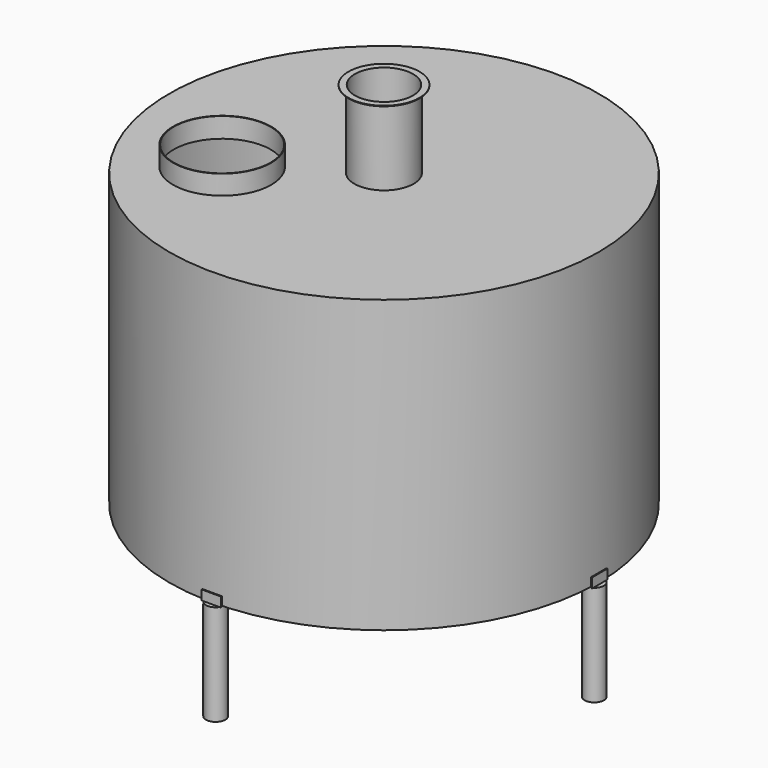
from build123d import *

# Parameters (mm, degrees)
F0_R      = 1106.75
F0_R_2    = 1103.75
F1_DEPTH  = 1500
F2_R      = 1103.75
F3_DEPTH  = 3
F4_R      = 1103.75
F4_R_2    = 250
F4_R_3    = 150
F5_DEPTH  = 3
F6_R      = 253
F6_R_2    = 250
F7_DEPTH  = 100
F8_R      = 153
F8_R_2    = 150
F9_DEPTH  = 400
F10_R     = 183
F10_R_2   = 150
F11_DEPTH = 3
F13_W     = 100
F13_H     = 50
F14_DEPTH = 5
F15_W     = 100
F15_H     = 5
F16_DEPTH = 50
F18_W     = 100
F18_H     = 50
F19_DEPTH = 5
F20_W     = 100
F20_H     = 5
F21_DEPTH = 50
F23_W     = 100
F23_H     = 50
F24_DEPTH = 5
F25_W     = 100
F25_H     = 5
F26_DEPTH = 50
F28_W     = 100
F28_H     = 50
F29_DEPTH = 5
F30_W     = 100
F30_H     = 5
F31_DEPTH = 50
F32_R     = 50
F33_DEPTH = 520
F34_R     = 50
F35_DEPTH = 520
F36_R     = 50
F37_DEPTH = 520
F38_R     = 50
F39_DEPTH = 520


with BuildPart() as f1:
    # F0 (on Top) → F1 (new body)
    with BuildSketch(Plane.XY):
        Circle(F0_R)
        Circle(F0_R_2, mode=Mode.SUBTRACT)
    extrude(amount=-F1_DEPTH)

    # F2 (on face) → F3 (join)
    with BuildSketch(Plane(origin=(0, 0, -1500), x_dir=(1, 0, 0), z_dir=(0, 0, -1))):
        Circle(F2_R)
    extrude(amount=-F3_DEPTH)

    # F4 (on face) → F5 (join)
    with BuildSketch(Plane.XY):
        Circle(F4_R)
        with Locations((-542.2929684516, -365.1128577139)):
            Circle(F4_R_2, mode=Mode.SUBTRACT)
        Circle(F4_R_3, mode=Mode.SUBTRACT)
    extrude(amount=-F5_DEPTH)

    # F6 (on face) → F7 (join)
    with BuildSketch(Plane.XY):
        with Locations((-542.2929684516, -365.1128577139)):
            Circle(F6_R)
        with Locations((-542.2929684516, -365.1128577139)):
            Circle(F6_R_2, mode=Mode.SUBTRACT)
    extrude(amount=F7_DEPTH)

    # F8 (on face) → F9 (join)
    with BuildSketch(Plane.XY):
        Circle(F8_R)
        Circle(F8_R_2, mode=Mode.SUBTRACT)
    extrude(amount=F9_DEPTH)

    # F10 (on face) → F11 (join)
    with BuildSketch(Plane.XY.offset(400)):
        Circle(F10_R)
        Circle(F10_R_2, mode=Mode.SUBTRACT)
    extrude(amount=-F11_DEPTH)


with BuildPart() as f14:
    # F13 (on offset) → F14 (new body)
    with BuildSketch(Plane.XZ.offset(1107.2876)):
        with Locations((0, -1480)):
            Rectangle(F13_W, F13_H)
    extrude(amount=F14_DEPTH)

    # F15 (on face) → F16 (join)
    with BuildSketch(Plane(origin=(0, -1107.2876, 0), x_dir=(-1, 0, 0), z_dir=(0, 1, 0))):
        with Locations((0, -1502.5)):
            Rectangle(F15_W, F15_H)
    extrude(amount=F16_DEPTH)

    # F36 (on face) → F37 (join)
    with BuildSketch(Plane(origin=(0, 0, -1505), x_dir=(1, 0, 0), z_dir=(0, 0, -1))):
        with Locations((0, 1084.7876)):
            Circle(F36_R)
    extrude(amount=F37_DEPTH)


with BuildPart() as f19:
    # F18 (on offset) → F19 (new body)
    with BuildSketch(Plane.XZ.offset(-1106.75031)):
        with Locations((0, -1480)):
            Rectangle(F18_W, F18_H)
    extrude(amount=-F19_DEPTH)

    # F20 (on face) → F21 (join)
    with BuildSketch(Plane.XZ.offset(-1106.75031)):
        with Locations((0, -1502.5)):
            Rectangle(F20_W, F20_H)
    extrude(amount=F21_DEPTH)

    # F32 (on face) → F33 (join)
    with BuildSketch(Plane(origin=(0, 0, -1505), x_dir=(1, 0, 0), z_dir=(0, 0, -1))):
        with Locations((0, -1084.25031)):
            Circle(F32_R)
    extrude(amount=F33_DEPTH)


with BuildPart() as f24:
    # F23 (on offset) → F24 (new body)
    with BuildSketch(Plane.YZ.offset(1106.75011)):
        with Locations((0, -1480)):
            Rectangle(F23_W, F23_H)
    extrude(amount=F24_DEPTH)

    # F25 (on face) → F26 (join)
    with BuildSketch(Plane(origin=(1106.75011, 0, 0), x_dir=(0, -1, 0), z_dir=(-1, 0, 0))):
        with Locations((0, -1502.5)):
            Rectangle(F25_W, F25_H)
    extrude(amount=F26_DEPTH)

    # F34 (on face) → F35 (join)
    with BuildSketch(Plane(origin=(0, 0, -1505), x_dir=(1, 0, 0), z_dir=(0, 0, -1))):
        with Locations((1084.25011, 0)):
            Circle(F34_R)
    extrude(amount=F35_DEPTH)


with BuildPart() as f29:
    # F28 (on offset) → F29 (new body)
    with BuildSketch(Plane.YZ.offset(-1106.75011)):
        with Locations((0, -1480)):
            Rectangle(F28_W, F28_H)
    extrude(amount=-F29_DEPTH)


with BuildPart() as f31:
    # F30 (on face) → F31 (new body)
    with BuildSketch(Plane.YZ.offset(-1106.75011)):
        with Locations((0, -1502.5)):
            Rectangle(F30_W, F30_H)
    extrude(amount=F31_DEPTH)

    # F38 (on face) → F39 (join)
    with BuildSketch(Plane(origin=(0, 0, -1505), x_dir=(1, 0, 0), z_dir=(0, 0, -1))):
        with Locations((-1081.75011, 0)):
            Circle(F38_R)
    extrude(amount=F39_DEPTH)


solid = Compound([f1.part, f14.part, f19.part, f24.part, f29.part, f31.part])
